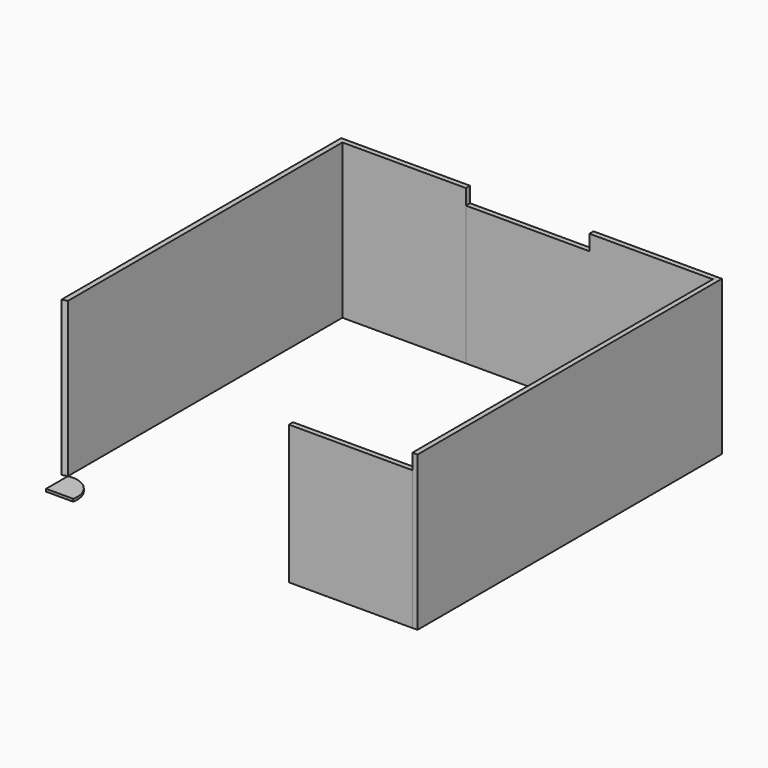
from build123d import *

# Parameters (mm, degrees)
F1_DEPTH = 1371.6
F0_W     = 1219.2
F0_H     = 50.8188946724
F2_DEPTH = 1371.6
F3_DEPTH = 1524
F4_DEPTH = 1524
F5_DEPTH = 1524
F6_DEPTH = 25.4


# Not quite as in the source:
# - ends of sketch curves that miss each other by under 0.0002 mm in the source are joined


with BuildPart() as f1:
    # F0 (on Top) → F1 (new body)
    with BuildSketch(Plane.XY):
        Polygon((3657.6, 0), (2438.3381043434, 0), (2438.3381043434, -50.7811053276), (3657.5381043434, -50.7811053276), align=None)
    extrude(amount=F1_DEPTH)


with BuildPart() as f2:
    # F0 (on Top) → F2 (new body)
    with BuildSketch(Plane.XY):
        with Locations((1828.8, 3683.0094473362)):
            Rectangle(F0_W, F0_H)
    extrude(amount=F2_DEPTH)

    # F0 (on Top) → F3 (join)
    with BuildSketch(Plane.XY):
        with Locations((3048, 3683.0094473362)):
            Rectangle(F0_W, F0_H)
    extrude(amount=F3_DEPTH)


with BuildPart() as f4:
    # F0 (on Top) → F4 (new body)
    with BuildSketch(Plane.XY):
        with BuildLine():
            ThreePointArc((-52.2567629814, 252.7961764093), (-26.6377838889, 262.8216290531), (0, 269.6969661319))
            Line((0, 269.6969661319), (0, 3657.6))
            Line((0, 3657.6), (1219.2, 3657.6))
            Line((1219.2, 3657.6), (1219.2, 3708.4188946724))
            Line((1219.2, 3708.4188946724), (-52.2567629814, 3708.4188946724))
            Line((-52.2567629814, 3708.4188946724), (-52.2567629814, 252.7961764093))
        make_face()
    extrude(amount=F4_DEPTH)


with BuildPart() as f5:
    # F0 (on Top) → F5 (new body)
    with BuildSketch(Plane.XY):
        Polygon((3657.6, 0.0188946724), (3657.6, 0), (3657.5381043434, -50.7811053276), (3708.3380666361, -50.8430009382), (3706.9432370186, 3708.4188946724), (3657.6, 3708.4188946724), (3657.6, 3657.6), align=None)
    extrude(amount=F5_DEPTH)


with BuildPart() as f6:
    # F0 (on Top) → F6 (new body)
    with BuildSketch(Plane.XY):
        with BuildLine():
            Line((0, 269.6969661319), (0, 0))
            Line((0, 0), (267.7718077733, 0))
            ThreePointArc((267.7718077733, 0), (271.1711559173, 22.5439223267), (272.3080413103, 45.3143306077))
            ThreePointArc((272.3080413103, 45.3143306077), (189.0804970171, 221.7365772824), (0, 269.6969661319))
        make_face()
    extrude(amount=-F6_DEPTH)


solid = Compound([f1.part, f2.part, f4.part, f5.part, f6.part])
